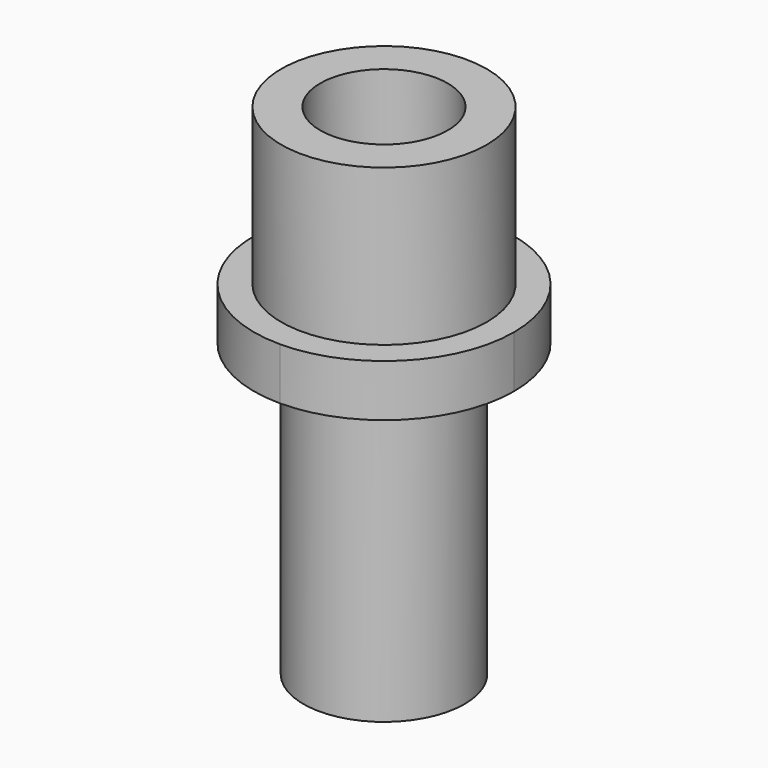
from build123d import *

# Parameters (mm, degrees)
F1_DEPTH = 30
F2_R     = 15.5
F2_R_2   = 12.25
F3_DEPTH = 66
F5_DEPTH = 10


# Not quite as in the source:
# - a feature names something its author has since deleted; it is built from what else it names


with BuildPart() as f1:
    # F0 (on Top) → F1 (new body)
    with BuildSketch(Plane.XY):
        with BuildLine():
            ThreePointArc((-19.75, 0), (0, -19.75), (19.75, 0))
            ThreePointArc((19.75, 0), (0, 19.75), (-19.75, 0))
        make_face()
        with BuildLine():
            ThreePointArc((12.25, 0), (0, -12.25), (-12.25, 0))
            ThreePointArc((-12.25, 0), (0, 12.25), (12.25, 0))
        make_face(mode=Mode.SUBTRACT)
    extrude(amount=F1_DEPTH)

    # F2 (on Top) → F3 (join)
    with BuildSketch(Plane.XY):
        Circle(F2_R)
        Circle(F2_R_2, mode=Mode.SUBTRACT)
    extrude(amount=-F3_DEPTH)

    # F4 (on Top) → F5 (join)
    with BuildSketch(Plane.XY):
        with BuildLine():
            ThreePointArc((0, -25), (17.6776695297, -17.6776695297), (25, 0))
            ThreePointArc((25, 0), (-17.6776695297, 17.6776695297), (0, -25))
        make_face()
        with BuildLine():
            ThreePointArc((12.25, 0), (8.6620580695, -8.6620580695), (0, -12.25))
            ThreePointArc((0, -12.25), (-8.6620580695, 8.6620580695), (12.25, 0))
        make_face(mode=Mode.SUBTRACT)
    extrude(amount=-F5_DEPTH)


solid = f1.part
